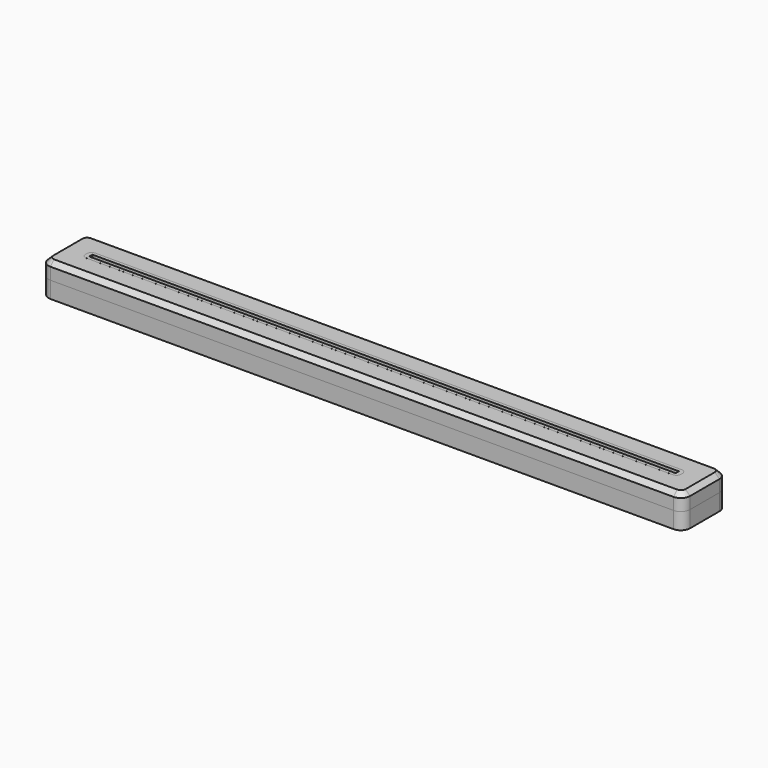
from build123d import *

# Parameters (mm, degrees)
F0_W      = 700
F0_H      = 60
F1_DEPTH  = 18
F2_DEPTH  = 18
F3_R      = 10
F3_2_R    = 10
F4_SIZE   = 5
F5_W      = 650
F5_H      = 12
F6_DEPTH  = 4.4
F7_R      = 5
F9_DEPTH  = 25
F11_DEPTH = 12
F12_W     = 200
F12_H     = 25
F13_DEPTH = 25
F14_R     = 5
F15_R     = 4
F16_DEPTH = 3
F17_W     = 640
F17_H     = 4.4
F18_DEPTH = 4.425
F19_R     = 1.5
F19_R_2   = 2
F20_DEPTH = 2.5
F21_R     = 2
F22_DEPTH = 1
F23_R     = 1.75
F24_DEPTH = 5
F25_W     = 176
F25_H     = 84.6484244061
F26_DEPTH = 25
F27_R     = 2


# Not quite as in the source:
# - ends of sketch curves that miss each other by under 0.0002 mm in the source are joined


with BuildPart() as f1:
    # F0 (on Top) → F1 (new body)
    with BuildSketch(Plane.XY):
        Rectangle(F0_W, F0_H)
    extrude(amount=F1_DEPTH)


with BuildPart() as f2:
    # F2 (new): a face of the model
    f2_faces = [f1.part.faces().sort_by_distance(p)[0] for p in [
        (0, 0, 18),
    ]]
    extrude(f2_faces, amount=F2_DEPTH)

    # F3#2
    f3_2_edges = [f2.edges().sort_by_distance(p)[0] for p in [
        (-350, -30, 27),
        (350, -30, 27),
        (350, 30, 27),
        (-350, 30, 27),
    ]]
    fillet(f3_2_edges, radius=F3_2_R)

    # F4
    f4_edges = [f2.edges().sort_by_distance(p)[0] for p in [
        (0, 30, 36),
        (350, 0, 36),
        (347.071068, -27.071068, 36),
        (347.071068, 27.071068, 36),
        (0, -30, 36),
        (-347.071068, -27.071068, 36),
        (-347.071068, 27.071068, 36),
        (-350, 0, 36),
    ]]
    chamfer(f4_edges, length=F4_SIZE)

    # F5 (on face) → F6 (cut)
    with BuildSketch(Plane.XY.offset(36)):
        Rectangle(F5_W, F5_H)
    extrude(amount=-F6_DEPTH, mode=Mode.SUBTRACT)

    # F7
    f7_edges = [f2.edges().sort_by_distance(p)[0] for p in [
        (-325, 6, 33.8),
        (-325, -6, 33.8),
        (325, 6, 33.8),
        (325, -6, 33.8),
    ]]
    fillet(f7_edges, radius=F7_R)


with BuildPart() as f1_1:
    add(f1.part)

    # F3
    f3_edges = [f1_1.edges().sort_by_distance(p)[0] for p in [
        (-350, -30, 9),
        (350, -30, 9),
        (350, 30, 9),
        (-350, 30, 9),
    ]]
    fillet(f3_edges, radius=F3_R)


with BuildPart() as f9_tool:
    # F8 (on face) → F9 (new body)
    with BuildSketch(Plane.XY.offset(31.6)):
        with BuildLine():
            Line((320, 3), (-320, 3))
            ThreePointArc((-320, 3), (-321.4142135624, 2.4142135624), (-322, 1))
            Line((-322, 1), (-322, -1))
            ThreePointArc((-322, -1), (-321.4142135624, -2.4142135624), (-320, -3))
            Line((-320, -3), (320, -3))
            ThreePointArc((320, -3), (321.4142135624, -2.4142135624), (322, -1))
            Line((322, -1), (322, 1))
            ThreePointArc((322, 1), (321.4142135624, 2.4142135624), (320, 3))
        make_face()
    extrude(amount=-F9_DEPTH)


with BuildPart() as f1_2:
    add(f1_1.part)

    # F9: cut by f9_tool
    add(f9_tool.part, mode=Mode.SUBTRACT)

    # F10 (on face) → F11 (cut)
    with BuildSketch(Plane.XY.offset(18)):
        with BuildLine():
            Line((-342, 20), (-342, -20))
            ThreePointArc((-342, -20), (-341.4142135624, -21.4142135624), (-340, -22))
            Line((-340, -22), (340, -22))
            ThreePointArc((340, -22), (341.4142135624, -21.4142135624), (342, -20))
            Line((342, -20), (342, 20))
            ThreePointArc((342, 20), (341.4142135624, 21.4142135624), (340, 22))
            Line((340, 22), (-340, 22))
            ThreePointArc((-340, 22), (-341.4142135624, 21.4142135624), (-342, 20))
        make_face()
    extrude(amount=-F11_DEPTH, mode=Mode.SUBTRACT)

    # F12 (on face) → F13 (cut)
    with BuildSketch(Plane.XY.offset(6)):
        Rectangle(F12_W, F12_H)
    extrude(amount=-F13_DEPTH, mode=Mode.SUBTRACT)

    # F14
    f14_edges = [f1_2.edges().sort_by_distance(p)[0] for p in [
        (100, 12.5, 3),
        (100, -12.5, 3),
        (-100, -12.5, 3),
        (-100, 12.5, 3),
    ]]
    fillet(f14_edges, radius=F14_R)

    # F15 (on face) → F16 (cut)
    with BuildSketch(Plane.XY.offset(6)):
        with Locations((-225, -10)):
            Circle(F15_R)
        with Locations((-225, 10)):
            Circle(F15_R)
        with Locations((-160, 10)):
            Circle(F15_R)
        with Locations((-160, -10)):
            Circle(F15_R)
        with Locations((-290, 10)):
            Circle(F15_R)
        with Locations((-290, -10)):
            Circle(F15_R)
        with Locations((290, -10)):
            Circle(F15_R)
        with Locations((160, 10)):
            Circle(F15_R)
        with Locations((225, 10)):
            Circle(F15_R)
        with Locations((225, -10)):
            Circle(F15_R)
        with Locations((290, 10)):
            Circle(F15_R)
        with Locations((160, -10)):
            Circle(F15_R)
    extrude(amount=-F16_DEPTH, mode=Mode.SUBTRACT)


with BuildPart() as f2_1:
    add(f2.part)

    # F9: cut by f9_tool
    add(f9_tool.part, mode=Mode.SUBTRACT)


with BuildPart() as f18:
    # F17 (on face) → F18 (new body)
    with BuildSketch(Plane.XY.offset(31.6)):
        with BuildLine():
            Line((320, 6), (-320, 6))
            ThreePointArc((-320, 6), (-323.5355339059, 4.5355339059), (-325, 1))
            Line((-325, 1), (-325, -1))
            ThreePointArc((-325, -1), (-323.5355339059, -4.5355339059), (-320, -6))
            Line((-320, -6), (320, -6))
            ThreePointArc((320, -6), (323.5355339059, -4.5355339059), (325, -1))
            Line((325, -1), (325, 1))
            ThreePointArc((325, 1), (323.5355339059, 4.5355339059), (320, 6))
        make_face()
        Rectangle(F17_W, F17_H, mode=Mode.SUBTRACT)
    extrude(amount=F18_DEPTH)


with BuildPart() as f20:
    # F19 (on face) → F20 (new body)
    with BuildSketch(Plane.XY.offset(6)):
        with BuildLine():
            ThreePointArc((-95, 18.5), (-102.7781745931, 15.2781745931), (-106, 7.5))
            Line((-106, 7.5), (-106, -7.5))
            ThreePointArc((-106, -7.5), (-102.7781745931, -15.2781745931), (-95, -18.5))
            Line((-95, -18.5), (95, -18.5))
            ThreePointArc((95, -18.5), (102.7781745931, -15.2781745931), (106, -7.5))
            Line((106, -7.5), (106, 7.5))
            ThreePointArc((106, 7.5), (102.7781745931, 15.2781745931), (95, 18.5))
            Line((95, 18.5), (-95, 18.5))
        make_face()
        with Locations((-93, -16)):
            Circle(F19_R, mode=Mode.SUBTRACT)
        with Locations((-25, -16)):
            Circle(F19_R, mode=Mode.SUBTRACT)
        with Locations((-93.5, -7.5)):
            Circle(F19_R_2, mode=Mode.SUBTRACT)
        with Locations((93, -16)):
            Circle(F19_R, mode=Mode.SUBTRACT)
        with Locations((93.5, -7.5)):
            Circle(F19_R_2, mode=Mode.SUBTRACT)
        with Locations((-103, 0)):
            Circle(F19_R, mode=Mode.SUBTRACT)
        with Locations((-93.5, 7.5)):
            Circle(F19_R_2, mode=Mode.SUBTRACT)
        with Locations((-93, 16)):
            Circle(F19_R, mode=Mode.SUBTRACT)
        with Locations((-25, 16)):
            Circle(F19_R, mode=Mode.SUBTRACT)
        with BuildLine():
            ThreePointArc((-88, 8.5), (-87.4142135624, 9.9142135624), (-86, 10.5))
            Line((-86, 10.5), (86, 10.5))
            ThreePointArc((86, 10.5), (87.4142135624, 9.9142135624), (88, 8.5))
            Line((88, 8.5), (88, -8.5))
            ThreePointArc((88, -8.5), (87.4142135624, -9.9142135624), (86, -10.5))
            Line((86, -10.5), (-86, -10.5))
            ThreePointArc((-86, -10.5), (-87.4142135624, -9.9142135624), (-88, -8.5))
            Line((-88, -8.5), (-88, 8.5))
        make_face(mode=Mode.SUBTRACT)
        with Locations((103, 0)):
            Circle(F19_R, mode=Mode.SUBTRACT)
        with Locations((93.5, 7.5)):
            Circle(F19_R_2, mode=Mode.SUBTRACT)
        with Locations((25, 16)):
            Circle(F19_R, mode=Mode.SUBTRACT)
        with Locations((93, 16)):
            Circle(F19_R, mode=Mode.SUBTRACT)
    extrude(amount=F20_DEPTH)

    # F21 (on face) → F22 (join)
    with BuildSketch(Plane(origin=(0, 0, 6), x_dir=(1, 0, 0), z_dir=(0, 0, -1))):
        with BuildLine():
            Line((-99.5, 7.5), (-99.5, -7.5))
            ThreePointArc((-99.5, -7.5), (-98.1819805153, -10.6819805153), (-95, -12))
            Line((-95, -12), (95, -12))
            ThreePointArc((95, -12), (98.1819805153, -10.6819805153), (99.5, -7.5))
            Line((99.5, -7.5), (99.5, 7.5))
            ThreePointArc((99.5, 7.5), (98.1819805153, 10.6819805153), (95, 12))
            Line((95, 12), (-95, 12))
            ThreePointArc((-95, 12), (-98.1819805153, 10.6819805153), (-99.5, 7.5))
        make_face()
        with Locations((-93.5, -7.5)):
            Circle(F21_R, mode=Mode.SUBTRACT)
        with Locations((93.5, -7.5)):
            Circle(F21_R, mode=Mode.SUBTRACT)
        with BuildLine():
            Line((-88.0000001416, -8.5), (-88.0000001416, 8.5))
            ThreePointArc((-88.0000001416, 8.5), (-87.4142134623, 9.9142134623), (-86, 10.4999998584))
            Line((-86, 10.4999998584), (86, 10.5000001416))
            ThreePointArc((86, 10.5000001416), (87.4142134623, 9.9142134623), (87.9999998584, 8.5))
            Line((87.9999998584, 8.5), (88.0000001416, -8.5))
            ThreePointArc((88.0000001416, -8.5), (87.4142134623, -9.9142134623), (86, -10.4999998584))
            Line((86, -10.4999998584), (-86, -10.5000001416))
            ThreePointArc((-86, -10.5000001416), (-87.4142134623, -9.9142134623), (-88.0000001416, -8.5))
        make_face(mode=Mode.SUBTRACT)
        with Locations((-93.5, 7.5)):
            Circle(F21_R, mode=Mode.SUBTRACT)
        with Locations((93.5, 7.5)):
            Circle(F21_R, mode=Mode.SUBTRACT)
    extrude(amount=F22_DEPTH)

    # F25 (on face) → F26 (cut)
    with BuildSketch(Plane.XY.offset(8.5)):
        Rectangle(F25_W, F25_H)
    extrude(amount=-F26_DEPTH, mode=Mode.SUBTRACT)

    # F27
    f27_edges = [f20.edges().sort_by_distance(p)[0] for p in [
        (-88, 18.5, 7.25),
        (-88, -18.5, 7.25),
    ]]
    fillet(f27_edges, radius=F27_R)


with BuildPart() as f24:
    # F23 (on face) → F24 (new body)
    with BuildSketch(Plane(origin=(0, 0, 5), x_dir=(1, 0, 0), z_dir=(0, 0, -1))):
        with BuildLine():
            ThreePointArc((-95, 12), (-98.1819805153, 10.6819805153), (-99.5, 7.5))
            Line((-99.5, 7.5), (-99.5, -7.5))
            ThreePointArc((-99.5, -7.5), (-98.1819805153, -10.6819805153), (-95, -12))
            Line((-95, -12), (95, -12))
            ThreePointArc((95, -12), (98.1819805153, -10.6819805153), (99.5, -7.5))
            Line((99.5, -7.5), (99.5, 7.5))
            ThreePointArc((99.5, 7.5), (98.1819805153, 10.6819805153), (95, 12))
            Line((95, 12), (-95, 12))
        make_face()
        with Locations((-93.5, -7.5)):
            Circle(F23_R, mode=Mode.SUBTRACT)
        with Locations((93.5, -7.5)):
            Circle(F23_R, mode=Mode.SUBTRACT)
        with Locations((-93.5, 7.5)):
            Circle(F23_R, mode=Mode.SUBTRACT)
        with Locations((93.5, 7.5)):
            Circle(F23_R, mode=Mode.SUBTRACT)
    extrude(amount=F24_DEPTH)


solid = Compound([f1_2.part, f2_1.part, f18.part, f20.part, f24.part])
